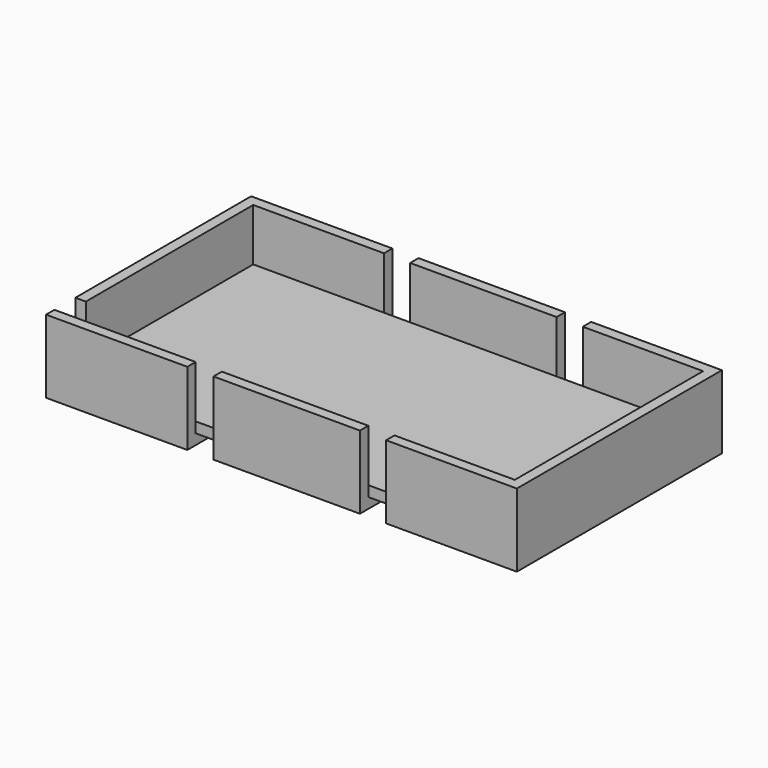
from build123d import *

# Parameters (mm, degrees)
F1_DEPTH = 2
F0_W     = 28.0000002682
F0_H     = 45
F0_H_2   = 2
F0_W_2   = 23
F0_W_3   = 4.9999997318
F0_W_4   = 5
F2_DEPTH = 2
F3_DEPTH = 12


with BuildPart() as f1:
    # F0 (on Top) → F1 (new body)
    with BuildSketch(Plane.XY):
        Polygon((-18, 22.5), (-43, 22.5), (-43, -17.5), (-43, -22.5), (-18, -22.5), align=None)
        Polygon((-18, -24.5), (-18, -22.5), (-43, -22.5), (-45, -22.5), (-45, -24.5), align=None)
        Polygon((-43, -17.5), (-43, 22.5), (-18, 22.5), (-18, 24.5), (-45, 24.5), (-45, -17.5), align=None)
    extrude(amount=-F1_DEPTH)



with BuildPart() as f1b:
    # F0 (on Top) → F1, piece 2 (new body)
    with BuildSketch(Plane.XY):
        with Locations((0.9999998659, 0)):
            Rectangle(F0_W, F0_H)
        with Locations((0.9999998659, -23.5)):
            Rectangle(F0_W, F0_H_2)
        with Locations((0.9999998659, 23.5)):
            Rectangle(F0_W, F0_H_2)
    extrude(amount=-F1_DEPTH)


with BuildPart() as f1c:
    # F0 (on Top) → F1, piece 3 (new body)
    with BuildSketch(Plane.XY):
        with Locations((31.5, 0)):
            Rectangle(F0_W_2, F0_H)
        Polygon((20, 24.5), (20, 22.5), (43, 22.5), (43, -22.5), (20, -22.5), (20, -24.5), (45, -24.5), (45, 24.5), align=None)
    extrude(amount=-F1_DEPTH)


with BuildPart() as f1_1:
    add(f1.part)

    add(f1b.part)  # F2 merges F1b

    add(f1c.part)  # F2 merges F1c
    # F0 (on Top) → F2 (join)
    with BuildSketch(Plane.XY):
        with Locations((31.5, 0)):
            Rectangle(F0_W_2, F0_H)
        with Locations((0.9999998659, 0)):
            Rectangle(F0_W, F0_H)
        Polygon((-18, 22.5), (-43, 22.5), (-43, -17.5), (-43, -22.5), (-18, -22.5), align=None)
        with Locations((-15.5000001341, 0)):
            Rectangle(F0_W_3, F0_H)
        with Locations((17.5, 0)):
            Rectangle(F0_W_4, F0_H)
    extrude(amount=F2_DEPTH)

    # F0 (on Top) → F3 (join)
    with BuildSketch(Plane.XY):
        Polygon((-43, -17.5), (-43, 22.5), (-18, 22.5), (-18, 24.5), (-45, 24.5), (-45, -17.5), align=None)
        Polygon((-18, -24.5), (-18, -22.5), (-43, -22.5), (-45, -22.5), (-45, -24.5), align=None)
        with Locations((0.9999998659, -23.5)):
            Rectangle(F0_W, F0_H_2)
        with Locations((0.9999998659, 23.5)):
            Rectangle(F0_W, F0_H_2)
        Polygon((20, 24.5), (20, 22.5), (43, 22.5), (43, -22.5), (20, -22.5), (20, -24.5), (45, -24.5), (45, 24.5), align=None)
    extrude(amount=F3_DEPTH)


solid = f1_1.part
